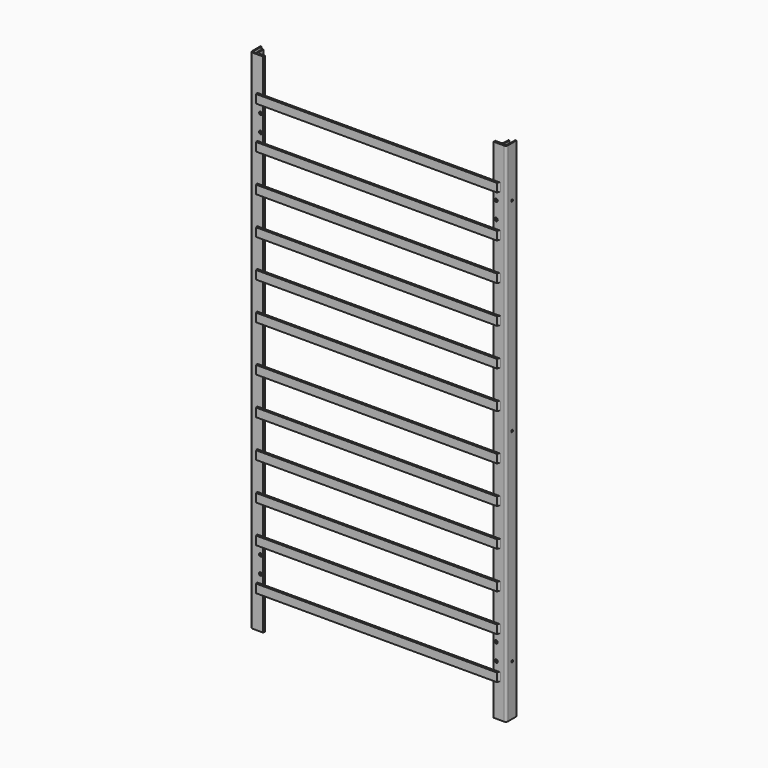
from build123d import *

# Parameters (mm, degrees)
F1_DEPTH      = 1524
F2_DEPTH      = 1524
F3_R          = 3.175
F4_DEPTH      = 384.176
F4_DEPTH_BACK = 384.176
F5_R          = 3.175
F7_DEPTH      = 38.101
F6_R          = 4.7625
F8_DEPTH      = 38.101
F9_W          = 723.9
F9_H          = 25.4
F10_DEPTH     = 6.35
F11_R         = 5.08


with BuildPart() as f1:
    # F0 (on Top) → F1 (new body)
    with BuildSketch(Plane.XY):
        with BuildLine():
            Line((-381, 0), (-384.175, 0))
            Line((-384.175, 0), (-384.175, -31.75))
            ThreePointArc((-384.175, -31.75), (-382.3151280605, -36.2401280605), (-377.825, -38.1))
            Line((-377.825, -38.1), (-346.075, -38.1))
            Line((-346.075, -38.1), (-346.075, -34.925))
            Line((-346.075, -34.925), (-365.125, -34.925))
            Line((-365.125, -34.925), (-374.65, -34.925))
            ThreePointArc((-374.65, -34.925), (-379.1401280605, -33.0651280605), (-381, -28.575))
            Line((-381, -28.575), (-381, 0))
        make_face()
    extrude(amount=F1_DEPTH)


with BuildPart() as f1b:
    # F0 (on Top) → F1, piece 2 (new body)
    with BuildSketch(Plane.XY):
        with BuildLine():
            Line((374.65, -34.925), (365.125, -34.925))
            Line((365.125, -34.925), (346.075, -34.925))
            Line((346.075, -34.925), (346.075, -38.1))
            Line((346.075, -38.1), (377.825, -38.1))
            ThreePointArc((377.825, -38.1), (382.3151280605, -36.2401280605), (384.175, -31.75))
            Line((384.175, -31.75), (384.175, 0))
            Line((384.175, 0), (381, 0))
            Line((381, 0), (381, -28.575))
            ThreePointArc((381, -28.575), (379.1401280605, -33.0651280605), (374.65, -34.925))
        make_face()
    extrude(amount=F1_DEPTH)


with BuildPart() as f2:
    # F0 (on Top) → F2 (new body)
    with BuildSketch(Plane.XY):
        with BuildLine():
            ThreePointArc((365.125, -34.925), (369.6151280605, -33.0651280605), (371.475, -28.575))
            Line((371.475, -28.575), (371.475, -9.525))
            Line((371.475, -9.525), (368.3, -9.525))
            Line((368.3, -9.525), (368.3, -25.4))
            ThreePointArc((368.3, -25.4), (366.4401280605, -29.8901280605), (361.95, -31.75))
            Line((361.95, -31.75), (346.075, -31.75))
            Line((346.075, -31.75), (346.075, -34.925))
            Line((346.075, -34.925), (365.125, -34.925))
        make_face()
    extrude(amount=F2_DEPTH)


with BuildPart() as f2b:
    # F0 (on Top) → F2, piece 2 (new body)
    with BuildSketch(Plane.XY):
        with BuildLine():
            Line((-365.125, -34.925), (-346.075, -34.925))
            Line((-346.075, -34.925), (-346.075, -31.75))
            Line((-346.075, -31.75), (-361.95, -31.75))
            ThreePointArc((-361.95, -31.75), (-366.4401280605, -29.8901280605), (-368.3, -25.4))
            Line((-368.3, -25.4), (-368.3, -9.525))
            Line((-368.3, -9.525), (-371.475, -9.525))
            Line((-371.475, -9.525), (-371.475, -28.575))
            ThreePointArc((-371.475, -28.575), (-369.6151280605, -33.0651280605), (-365.125, -34.925))
        make_face()
    extrude(amount=F2_DEPTH)


with BuildPart() as f4_tool:
    # F3 (on Right) → F4 (new body, two sides)
    with BuildSketch(Plane.YZ) as f4_sk:
        with Locations((-15.875, 152.4)):
            Circle(F3_R)
        with Locations((-15.875, 762)):
            Circle(F3_R)
        with Locations((-15.875, 1371.6)):
            Circle(F3_R)
    extrude(amount=-F4_DEPTH)
    extrude(f4_sk.sketch, amount=F4_DEPTH_BACK)


with BuildPart() as f1_1:
    add(f1.part)

    # F4: cut by f4_tool
    add(f4_tool.part, mode=Mode.SUBTRACT)


with BuildPart() as f1b_1:
    add(f1b.part)

    # F4: cut by f4_tool
    add(f4_tool.part, mode=Mode.SUBTRACT)


with BuildPart() as f7_tool:
    # F5 (on Front) → F7 (new body, through all)
    with BuildSketch(Plane.XZ):
        with Locations((-354.0125, 152.4)):
            Circle(F5_R)
        with Locations((-354.0125, 203.2)):
            Circle(F5_R)
        with Locations((-354.0125, 1320.8)):
            Circle(F5_R)
        with Locations((-354.0125, 1371.6)):
            Circle(F5_R)
        with Locations((354.0125, 152.4)):
            Circle(F5_R)
        with Locations((354.0125, 203.2)):
            Circle(F5_R)
        with Locations((354.0125, 1371.6)):
            Circle(F5_R)
        with Locations((354.0125, 1320.8)):
            Circle(F5_R)
    extrude(amount=F7_DEPTH)


with BuildPart() as f1_2:
    add(f1_1.part)

    # F7: cut by f7_tool
    add(f7_tool.part, mode=Mode.SUBTRACT)


with BuildPart() as f1b_2:
    add(f1b_1.part)

    # F7: cut by f7_tool
    add(f7_tool.part, mode=Mode.SUBTRACT)


with BuildPart() as f2_1:
    add(f2.part)

    # F7: cut by f7_tool
    add(f7_tool.part, mode=Mode.SUBTRACT)


with BuildPart() as f2b_1:
    add(f2b.part)

    # F7: cut by f7_tool
    add(f7_tool.part, mode=Mode.SUBTRACT)


with BuildPart() as f8_tool:
    # F6 (on Front) → F8 (new body, through all)
    with BuildSketch(Plane.XZ):
        with Locations((-354.0125, 1371.6)):
            Circle(F6_R)
        with Locations((-354.0125, 1320.8)):
            Circle(F6_R)
        with Locations((-354.0125, 203.2)):
            Circle(F6_R)
        with Locations((-354.0125, 152.4)):
            Circle(F6_R)
        with Locations((354.0125, 152.4)):
            Circle(F6_R)
        with Locations((354.0125, 203.2)):
            Circle(F6_R)
        with Locations((354.0125, 1371.6)):
            Circle(F6_R)
        with Locations((354.0125, 1320.8)):
            Circle(F6_R)
    extrude(amount=F8_DEPTH)


with BuildPart() as f1_3:
    add(f1_2.part)

    # F8: cut by f8_tool
    add(f8_tool.part, mode=Mode.SUBTRACT)



with BuildPart() as f1b_3:
    add(f1b_2.part)

    # F8: cut by f8_tool
    add(f8_tool.part, mode=Mode.SUBTRACT)


with BuildPart() as f1_4:
    add(f1_3.part)

    add(f1b_3.part)  # F10 merges F1b
    # F9 (on face) → F10 (join)
    with BuildSketch(Plane.XZ.offset(38.1)):
        with Locations((0, 1409.7)):
            Rectangle(F9_W, F9_H)
        with Locations((0, 1282.7)):
            Rectangle(F9_W, F9_H)
        with Locations((0, 1169.8111111111)):
            Rectangle(F9_W, F9_H)
        with Locations((0, 1056.9222222222)):
            Rectangle(F9_W, F9_H)
        with Locations((0, 944.0333333333)):
            Rectangle(F9_W, F9_H)
        with Locations((0, 831.1444444444)):
            Rectangle(F9_W, F9_H)
        with Locations((0, 467.0777777778)):
            Rectangle(F9_W, F9_H)
        with Locations((0, 579.9666666667)):
            Rectangle(F9_W, F9_H)
        with Locations((0, 114.3)):
            Rectangle(F9_W, F9_H)
        with Locations((0, 692.8555555556)):
            Rectangle(F9_W, F9_H)
        with Locations((0, 241.3)):
            Rectangle(F9_W, F9_H)
        with Locations((0, 354.1888888889)):
            Rectangle(F9_W, F9_H)
    extrude(amount=F10_DEPTH)

    # F11
    f11_edges = [f1_4.edges().sort_by_distance(p)[0] for p in [
        (361.95, -38.1, 1409.7),
        (361.95, -38.1, 1282.7),
        (361.95, -38.1, 1169.811111),
        (361.95, -38.1, 1056.922222),
        (361.95, -38.1, 944.033333),
        (361.95, -38.1, 831.144444),
        (361.95, -38.1, 692.855556),
        (361.95, -38.1, 579.966667),
        (361.95, -38.1, 467.077778),
        (361.95, -38.1, 354.188889),
        (361.95, -38.1, 241.3),
        (361.95, -38.1, 114.3),
        (-361.95, -38.1, 114.3),
        (-361.95, -38.1, 241.3),
        (-361.95, -38.1, 354.188889),
        (-361.95, -38.1, 467.077778),
        (-361.95, -38.1, 579.966667),
        (-361.95, -38.1, 692.855556),
        (-361.95, -38.1, 831.144444),
        (-361.95, -38.1, 944.033333),
        (-361.95, -38.1, 1056.922222),
        (-361.95, -38.1, 1169.811111),
        (-361.95, -38.1, 1282.7),
        (-361.95, -38.1, 1409.7),
    ]]
    fillet(f11_edges, radius=F11_R)


solid = Compound([f2_1.part, f2b_1.part, f1_4.part])
